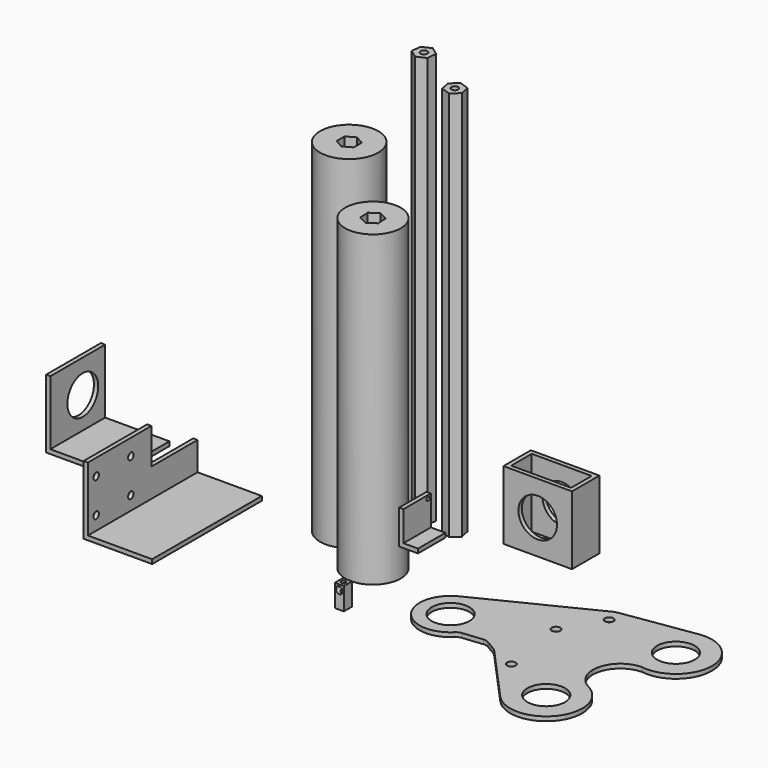
from build123d import *

# Parameters (mm, degrees)
F0_R      = 2.5527
F1_DEPTH  = 289.56
F2_DEPTH  = 304.8
F3_R      = 3.175
F3_R_2    = 13.97
F4_DEPTH  = 3.175
F5_R      = 21.59
F6_DEPTH  = 254
F7_R      = 20.6375
F8_DEPTH  = 228.6
F9_R      = 6.35
F10_W     = 50.8
F10_H     = 25.4
F10_W_2   = 44.45
F10_H_2   = 19.05
F11_DEPTH = 50.8
F12_R     = 14.2875
F13_DEPTH = 25.4
F15_DEPTH = 101.6
F16_R     = 2.5527
F16_W     = 42.781021446
F16_H     = 26.5406374857
F17_DEPTH = 3.175
F19_DEPTH = 25.4
F20_R     = 1.4067906503
F21_DEPTH = 3.175
F22_W     = 6.7378332439
F22_H     = 7.62
F22_R     = 1.778
F23_DEPTH = 16.51
F24_R     = 2.5527
F25_DEPTH = 7.62
F27_DEPTH = 50.8
F28_R     = 14.2875
F29_DEPTH = 25.4


# Not quite as in the source:
# - a feature names something its author has since deleted; it is built from what else it names


with BuildPart() as f1:
    # F0 (on Top) → F1 (new body)
    with BuildSketch(Plane.XY):
        Polygon((-49.7183075275, 43.0769950958), (-42.7458795893, 40.8079464007), (-37.2946118079, 45.7117217736), (-38.8157719646, 52.8845458417), (-45.7881999028, 55.1535945367), (-51.2394676842, 50.2498191638), align=None)
        with Locations((-44.267039746, 47.9807704687)):
            Circle(F0_R, mode=Mode.SUBTRACT)
    extrude(amount=F1_DEPTH)


with BuildPart() as f2:
    # F0 (on Top) → F2 (new body)
    with BuildSketch(Plane.XY):
        Polygon((-68.7933438248, 41.7760031993), (-62.1052457259, 44.7814444568), (-61.3639851549, 52.0762279422), (-67.3108226829, 56.3655701702), (-73.9989207819, 53.3601289127), (-74.7401813528, 46.0653454273), align=None)
        with Locations((-68.0520832539, 49.0707866848)):
            Circle(F0_R, mode=Mode.SUBTRACT)
    extrude(amount=F2_DEPTH)


with BuildPart() as f4:
    # F3 (on Top) → F4 (new body)
    with BuildSketch(Plane.XY):
        with BuildLine():
            ThreePointArc((140.9444579385, -59.8277957087), (130.5002323104, -37.0649228102), (150.0837722501, -21.4535425063))
            ThreePointArc((150.0837722501, -21.4535425063), (180.7781507554, 4.8935224463), (150.1184854314, 31.2809744958))
            Line((150.1184854314, 31.2809744958), (96.617753451, 23.1865048445))
            ThreePointArc((96.617753451, 23.1865048445), (95.0662956112, 22.8270454376), (93.588950484, 22.2323321711))
            Line((93.588950484, 22.2323321711), (11.8021475778, -18.3116541727))
            ThreePointArc((11.8021475778, -18.3116541727), (4.0028834206, -52.9454255019), (39.5004115999, -53.4475520253))
            Line((39.5004115999, -53.4475520253), (58.8957592845, -51.4868795872))
            Line((58.8957592845, -51.4868795872), (69.3466052871, -57.6993331615))
            Line((69.3466052871, -57.6993331615), (108.9380329404, -101.4256812442))
            ThreePointArc((108.9380329404, -101.4256812442), (132.4492727351, -109.9313966124), (152.6725834267, -95.2295839597))
            ThreePointArc((152.6725834267, -95.2295839597), (154.0250448726, -75.1379546349), (140.9444579385, -59.8277957087))
        make_face()
        with Locations((88.6054252238, -65.7030506208)):
            Circle(F3_R, mode=Mode.SUBTRACT)
        with Locations((128.7081565336, -83.5250915023)):
            Circle(F3_R_2, mode=Mode.SUBTRACT)
        with Locations((21.9553885414, -38.7931408847)):
            Circle(F3_R_2, mode=Mode.SUBTRACT)
        with Locations((81.5415307879, -15.4408300295)):
            Circle(F3_R, mode=Mode.SUBTRACT)
        with Locations((98.1559753418, 13.0195636302)):
            Circle(F3_R, mode=Mode.SUBTRACT)
        with Locations((154.1081565336, 4.9110783167)):
            Circle(F3_R_2, mode=Mode.SUBTRACT)
    extrude(amount=F4_DEPTH)

    # F9
    f9_edges = [f4.edges().sort_by_distance(p)[0] for p in [
        (108.938033, -101.425681, 1.5875),
        (39.500412, -53.447552, 1.5875),
        (58.895759, -51.48688, 1.5875),
        (69.346605, -57.699333, 1.5875),
    ]]
    fillet(f9_edges, radius=F9_R)


with BuildPart() as f6:
    # F5 (on Top) → F6 (new body)
    with BuildSketch(Plane.XY):
        with Locations((-92.7056819201, 10.6180952862)):
            Circle(F5_R)
        Polygon((-86.3578141646, 14.2879601737), (-86.3535518213, 6.9556129938), (-92.7014195768, 3.2857481063), (-99.0535496755, 6.9482303987), (-99.0578120188, 14.2805775786), (-92.7099442633, 17.950442466), align=None, mode=Mode.SUBTRACT)
    extrude(amount=F6_DEPTH)


with BuildPart() as f8:
    # F7 (on Top) → F8 (new body)
    with BuildSketch(Plane.XY):
        with Locations((-52.8326742351, -17.1844772995)):
            Circle(F7_R)
        Polygon((-46.699447393, -13.1661615035), (-46.2860972543, -20.4868496539), (-52.4193240964, -24.5051654499), (-58.9659010772, -21.2027930955), (-59.3792512159, -13.882104945), (-53.2460243738, -9.863789149), align=None, mode=Mode.SUBTRACT)
    extrude(amount=F8_DEPTH)


with BuildPart() as f11:
    # F10 (on Top) → F11 (new body)
    with BuildSketch(Plane.XY):
        with Locations((12.4985007569, 66.5276864394)):
            Rectangle(F10_W, F10_H)
        with Locations((12.4985007569, 66.5276864394)):
            Rectangle(F10_W_2, F10_H_2, mode=Mode.SUBTRACT)
    extrude(amount=F11_DEPTH)

    # F12 (on face) → F13 (cut, through all)
    with BuildSketch(Plane(origin=(0, 79.2276864394, 0), x_dir=(-1, 0, 0), z_dir=(0, 1, 0))):
        with Locations((-12.4985007569, 25.4)):
            Circle(F12_R)
    extrude(amount=-F13_DEPTH, mode=Mode.SUBTRACT)


with BuildPart() as f15:
    # F14 (on Front) → F15 (new body)
    with BuildSketch(Plane.XZ):
        Polygon((-196.6332101345, 56.52981406), (-199.8082101345, 56.52981406), (-199.8082101345, 5.72981406), (-149.0082101345, 5.72981406), (-149.0082101345, 8.90481406), (-196.6332101345, 8.90481406), align=None)
    extrude(amount=F15_DEPTH)

    # F16 (on face) → F17 (cut, through all)
    with BuildSketch(Plane.YZ.offset(-196.6332101345)):
        with Locations((-93.98, 44.46481406)):
            Circle(F16_R)
        with Locations((-93.98, 19.06481406)):
            Circle(F16_R)
        with Locations((-61.849, 19.06481406)):
            Circle(F16_R)
        with Locations((-61.849, 44.46481406)):
            Circle(F16_R)
        with Locations((-21.390510723, 43.2594953172)):
            Rectangle(F16_W, F16_H)
    extrude(amount=-F17_DEPTH, mode=Mode.SUBTRACT)


with BuildPart() as f19:
    # F18 (on Front) → F19 (new body)
    with BuildSketch(Plane.XZ):
        Polygon((-23.6719425689, 51.3674189275), (-26.8469425689, 51.3674189275), (-26.8469425689, 25.9674189275), (-12.8769425689, 25.9674189275), (-12.8769425689, 29.1424189275), (-23.6719425689, 29.1424189275), align=None)
    extrude(amount=F19_DEPTH)

    # F20 (on face) → F21 (cut, through all)
    with BuildSketch(Plane.YZ.offset(-23.6719425689)):
        with Locations((-2.615345642, 48.8274189275)):
            Circle(F20_R)
    extrude(amount=-F21_DEPTH, mode=Mode.SUBTRACT)


with BuildPart() as f23:
    # F22 (on Top) → F23 (new body)
    with BuildSketch(Plane.XY):
        with Locations((-35.5452783406, -66.1711778778)):
            Rectangle(F22_W, F22_H)
        with Locations((-35.5452783406, -66.1711778778)):
            Circle(F22_R, mode=Mode.SUBTRACT)
    extrude(amount=F23_DEPTH)

    # F24 (on face) → F25 (cut, through all)
    with BuildSketch(Plane.XZ.offset(69.9811778778)):
        with Locations((-35.5452783406, 12.6873)):
            Circle(F24_R)
    extrude(amount=-F25_DEPTH, mode=Mode.SUBTRACT)


with BuildPart() as f27:
    # F26 (on Front) → F27 (new body)
    with BuildSketch(Plane.XZ):
        Polygon((-265.1258880146, 69.9299412084), (-268.3008880146, 69.9299412084), (-268.3008880146, 19.1299412084), (-217.5008880146, 19.1299412084), (-217.5008880146, 22.3049412084), (-265.1258880146, 22.3049412084), align=None)
    extrude(amount=F27_DEPTH)

    # F28 (on face) → F29 (cut)
    with BuildSketch(Plane(origin=(-268.3008880146, 0, 0), x_dir=(0, -1, 0), z_dir=(-1, 0, 0))):
        with Locations((20.7391, 45.4824412084)):
            Circle(F28_R)
    extrude(amount=-F29_DEPTH, mode=Mode.SUBTRACT)


solid = Compound([f1.part, f2.part, f4.part, f6.part, f8.part, f11.part, f15.part, f19.part, f23.part, f27.part])
